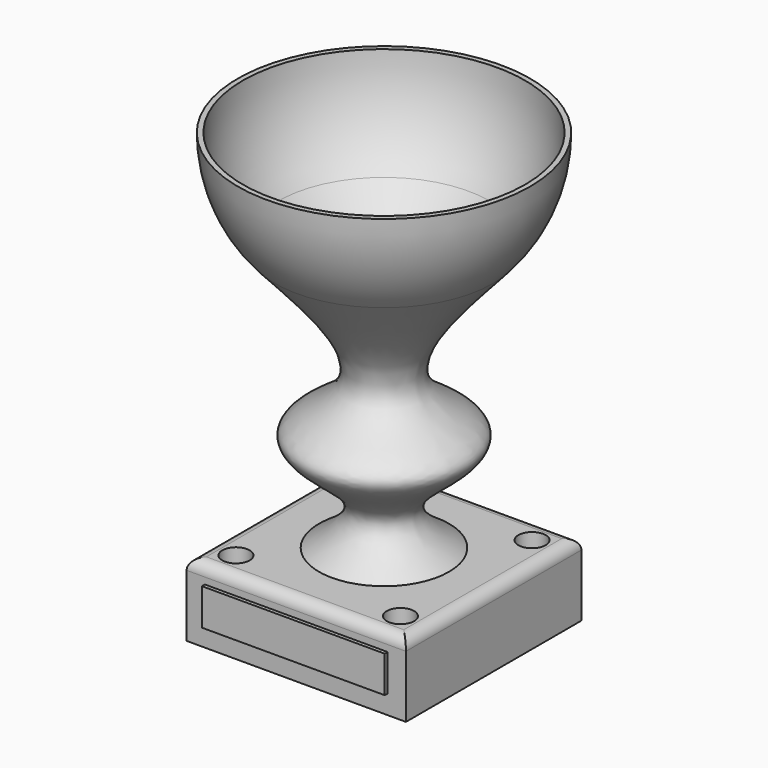
from build123d import *

# Parameters (mm, degrees)
F0_W      = 152.4
F0_H      = 152.4
F1_DEPTH  = 50.8
F2_W      = 127
F2_H      = 25.4
F3_DEPTH  = 2.54
F7_R      = 9.525
F8_DEPTH  = 110.236
F9_R      = 7.62
F11_DEPTH = 3.048


# Not quite as in the source:
# - ends of sketch curves that miss each other by under 0.0002 mm in the source are joined
# - the dataset's text gives a spline's control points without its knots; the knots are read off the source's solid


with BuildPart() as f1:
    # F0 (on Top) → F1 (new body)
    with BuildSketch(Plane.XY):
        Rectangle(F0_W, F0_H)
    extrude(amount=F1_DEPTH)

    # F7 (on face) → F8 (cut)
    with BuildSketch(Plane.XY.offset(50.8)):
        with Locations((-57.15, 57.15)):
            Circle(F7_R)
        with Locations((-57.15, -57.15)):
            Circle(F7_R)
        with Locations((57.15, 57.15)):
            Circle(F7_R)
        with Locations((57.15, -57.15)):
            Circle(F7_R)
    extrude(amount=-F8_DEPTH, mode=Mode.SUBTRACT)

    # F9
    f9_edges = [f1.edges().sort_by_distance(p)[0] for p in [
        (76.2, 0, 50.8),
        (0, -76.2, 50.8),
        (-76.2, 0, 50.8),
        (0, 76.2, 50.8),
    ]]
    fillet(f9_edges, radius=F9_R)

    # F10 (on face) → F11 (join)
    with BuildSketch(Plane(origin=(0, 0, 0), x_dir=(1, 0, 0), z_dir=(0, 0, -1))):
        with BuildLine():
            add(Edge.make_bspline(
                [(0, 7.7021815814), (-3.6313977016, 11.3563567366), (-3.1874263552, 69.6094998973), (7.4191084282, 38.7575716101), (6.4925414352, 26.570288192), (6.378028943, 20.1151630572), (5.6407833061, 14.3187155103), (1.4670161298, 6.2259637902), (0, 7.7021815814)],
                knots=[0, 0, 0, 0, 0.3055644832, 0.4718060515, 0.6473357636, 0.7554248666, 0.8765577162, 1, 1, 1, 1], degree=3))
        make_face()
    extrude(amount=F11_DEPTH)


with BuildPart() as f3:
    # F2 (on face) → F3 (new body)
    with BuildSketch(Plane.XZ.offset(76.2)):
        with Locations((0, 25.9362608194)):
            Rectangle(F2_W, F2_H)
    extrude(amount=F3_DEPTH)


with BuildPart() as f5:
    # F4 (on Front) → F5 (revolve)
    with BuildSketch(Plane.XZ):
        with BuildLine():
            add(Edge.make_bspline(
                [(75.661617229, 236.9923331894), (48.8089731412, 207.0294311443), (-7.0257436543, 149.6910017246), (86.3868939609, 121.984383041), (1.5417803268, 80.6547364845), (31.7099079405, 59.9084357565), (45.2254201298, 50.8)],
                knots=[0, 0, 0, 0, 0.3285576695, 0.5539276428, 0.7955188793, 0.9963286934, 0.9963286934, 0.9963286934, 0.9963286934], degree=3))
            ThreePointArc((75.661617229, 236.9923331894), (94.8940996861, 268.5002776214), (101.6, 304.8))
            Line((101.6, 304.8), (98.0440034793, 304.8))
            ThreePointArc((98.0440034793, 304.8), (91.5728094467, 269.7707666615), (73.013463217, 239.3655992057))
            add(Edge.make_bspline(
                [(73.013463217, 239.3655992057), (67.920107087, 233.6822955316), (59.9132388158, 224.9080810469), (49.5144766657, 213.0724037347), (42.1032033451, 204.2105349703), (35.3277167522, 195.4417614882), (29.4344187183, 186.8339328536), (24.6718429025, 178.4375490656), (21.861423182, 171.6329618437), (20.466524302, 166.2953857414), (19.8994522062, 162.3431593554), (19.8726484133, 158.4492168052), (20.3580838755, 155.2759809832), (21.0796156785, 152.8109495588), (21.6735647185, 151.3074471828), (22.2338100805, 150.1361963456), (22.842733407, 148.9961660864), (23.690444059, 147.6239675183), (24.8262738622, 146.0577918295), (26.4767272839, 144.0670223462), (28.7570911961, 141.7431065145), (31.7384693201, 139.1638771412), (35.9168668967, 135.9477858716), (40.2201747798, 132.9964903331), (44.2743051668, 130.2196745078), (47.0905525309, 128.213423825), (49.5788319814, 126.2805069174), (51.6306968123, 124.4358211831), (53.1405611374, 122.7235289983), (53.8846273606, 121.4873467256), (54.1985887401, 120.6586611694), (54.2990928501, 120.2014984584), (54.3330795674, 119.8544550371), (54.3368190338, 119.6004824772), (54.3180508606, 119.327979815), (54.2584026878, 118.9280529455), (54.1097510248, 118.3560271553), (53.682458921, 117.2866522567), (52.759520809, 115.7004483833), (51.0515992425, 113.5352300761), (48.8354897039, 111.200654216), (46.2130481373, 108.7502362484), (42.3100682686, 105.3718770838), (36.9165657046, 100.9958002819), (31.4630021414, 96.4988716584), (27.4167626018, 92.8394905445), (24.6243409961, 90.0554802307), (22.5681942263, 87.6859133637), (21.1298777686, 85.7382020612), (20.1676515107, 84.242551311), (19.4760032184, 82.957957537), (18.9996608274, 81.9023177267), (18.5785332228, 80.823579839), (18.1733147203, 79.4592117853), (17.7877032197, 77.2603933736), (17.8007080788, 74.5241503682), (18.5270440062, 71.3969331314), (19.8210652009, 68.483476961), (21.5600675308, 65.7654911851), (23.6587765867, 63.2011292819), (26.8550036618, 59.9361604346), (31.4692891324, 56.0687114488), (35.9738707918, 52.8204385731), (38.4831657072, 51.0841871883), (38.8961215908, 50.7999869925)],
                knots=[0, 0, 0, 0, 0.0625, 0.09375, 0.125, 0.15625, 0.1875, 0.21875, 0.25, 0.265625, 0.28125, 0.296875, 0.3125, 0.3203125, 0.328125, 0.33203125, 0.3359375, 0.34375, 0.3515625, 0.359375, 0.375, 0.390625, 0.40625, 0.4375, 0.453125, 0.46875, 0.484375, 0.5, 0.515625, 0.53125, 0.5390625, 0.546875, 0.55078125, 0.5546875, 0.55859375, 0.5625, 0.5703125, 0.578125, 0.59375, 0.609375, 0.625, 0.640625, 0.65625, 0.6875, 0.71875, 0.734375, 0.75, 0.765625, 0.7734375, 0.78125, 0.7890625, 0.79296875, 0.796875, 0.8046875, 0.8125, 0.828125, 0.84375, 0.859375, 0.875, 0.890625, 0.90625, 0.9375, 0.96875, 0.9748882231, 0.9748882231, 0.9748882231, 0.9748882231], degree=3))
            Line((38.8961215908, 50.7999869925), (45.2254201298, 50.8))
        make_face()
    revolve(axis=Axis((0, 0, 177.8), (0, 0, 1)))


solid = Compound([f1.part, f3.part, f5.part])
